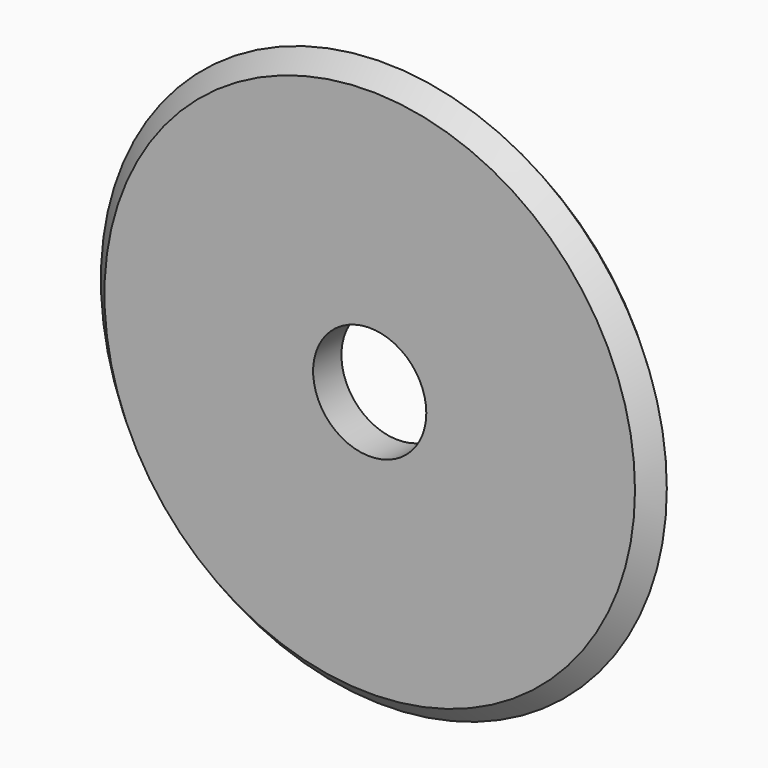
from build123d import *

# Parameters (mm, degrees)
F0_R     = 50.8
F0_R_2   = 10.16
F1_DEPTH = 6.35
F2_SIZE  = 3.175
F3_SIZE  = 3.17499


# Not quite as in the source:
# - a fillet or chamfer is up to 0.001 mm smaller than in the source, because OpenCascade refuses the exact size


with BuildPart() as f1:
    # F0 (on Front) → F1 (new body)
    with BuildSketch(Plane.XZ):
        Circle(F0_R)
        Circle(F0_R_2, mode=Mode.SUBTRACT)
    extrude(amount=F1_DEPTH)

    # F2
    f2_edges = [f1.edges().sort_by_distance(p)[0] for p in [
        (-50.8, -6.35, 0),
    ]]
    chamfer(f2_edges, length=F2_SIZE)

    # F3 (size 3.175 in the source; OpenCascade refuses exactly that, so slightly less here)
    f3_edges = [f1.edges().sort_by_distance(p)[0] for p in [
        (-50.8, 0, 0),
    ]]
    chamfer(f3_edges, length=F3_SIZE)


solid = f1.part
